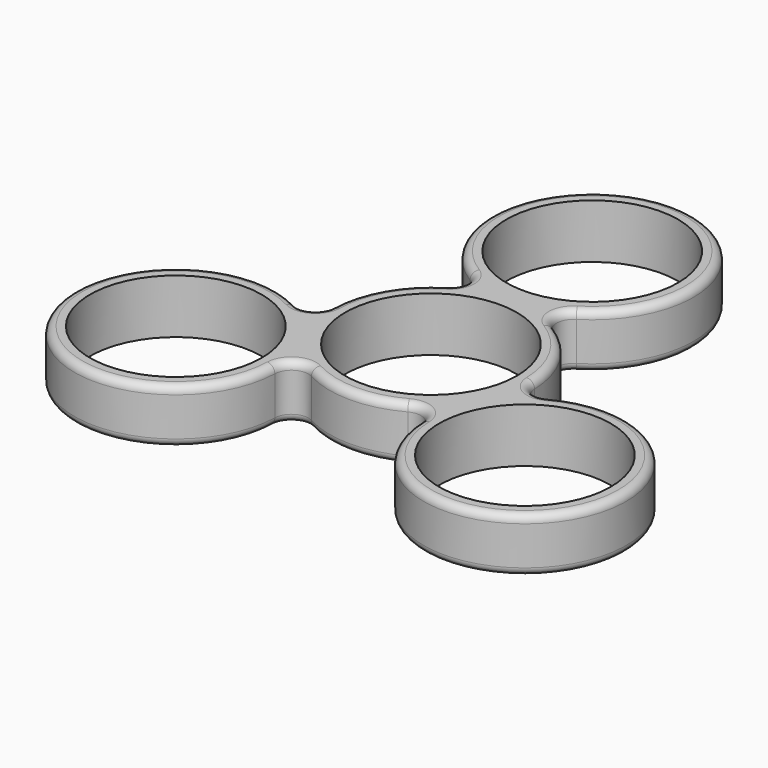
from build123d import *

# Parameters (mm, degrees)
F0_R     = 11.075
F1_DEPTH = 3.5
F2_R     = 1


# Not quite as in the source:
# - a feature names something its author has since deleted; it is built from what else it names


with BuildPart() as f1:
    # F0 (on Top) → F1 (new body, symmetric)
    with BuildSketch(Plane.XY):
        with BuildLine():
            ThreePointArc((6.8525738406, 11.1354324909), (0, 13.075), (-6.8525738406, 11.1354324909))
            ThreePointArc((-6.8525738406, 11.1354324909), (-11.3232821545, 6.5375), (-13.0698543395, 0.3667867818))
            ThreePointArc((-13.0698543395, 0.3667867818), (-11.3232821545, -6.5375), (-6.217280499, -11.5022192727))
            ThreePointArc((-6.217280499, -11.5022192727), (0, -13.075), (6.217280499, -11.5022192727))
            ThreePointArc((6.217280499, -11.5022192727), (8.3529990104, -11.5321813184), (9.4468061589, -13.3667867818))
            ThreePointArc((9.4468061589, -13.3667867818), (33.8399426529, -19.5375), (16.2993799994, -1.4977807273))
            ThreePointArc((16.2993799994, -1.4977807273), (14.163661488, -1.4678186816), (13.0698543395, 0.3667867818))
            ThreePointArc((13.0698543395, 0.3667867818), (11.3232821545, 6.5375), (6.8525738406, 11.1354324909))
        make_face()
        with Locations((22.5166604984, -13)):
            Circle(F0_R, mode=Mode.SUBTRACT)
        Circle(F0_R, mode=Mode.SUBTRACT)
        with BuildLine():
            ThreePointArc((-6.8525738406, 14.8645675091), (-5.8106624775, 13), (-6.8525738406, 11.1354324909))
            ThreePointArc((-6.8525738406, 11.1354324909), (0, 13.075), (6.8525738406, 11.1354324909))
            ThreePointArc((6.8525738406, 11.1354324909), (5.8106624775, 13), (6.8525738406, 14.8645675091))
            ThreePointArc((6.8525738406, 14.8645675091), (0, 39.075), (-6.8525738406, 14.8645675091))
        make_face()
        with Locations((0, 26)):
            Circle(F0_R, mode=Mode.SUBTRACT)
        with BuildLine():
            ThreePointArc((-6.217280499, -11.5022192727), (-11.3232821545, -6.5375), (-13.0698543395, 0.3667867818))
            ThreePointArc((-13.0698543395, 0.3667867818), (-14.163661488, -1.4678186816), (-16.2993799994, -1.4977807273))
            ThreePointArc((-16.2993799994, -1.4977807273), (-33.8399426529, -19.5375), (-9.4468061589, -13.3667867818))
            ThreePointArc((-9.4468061589, -13.3667867818), (-8.3529990104, -11.5321813184), (-6.217280499, -11.5022192727))
        make_face()
        with Locations((-22.5166604984, -13)):
            Circle(F0_R, mode=Mode.SUBTRACT)
    extrude(amount=F1_DEPTH, both=True)

    # F2
    f2_edges = [f1.edges().sort_by_distance(p)[0] for p in [
        (-14.163661, -1.467819, 3.5),
        (5.810662, 13, -3.5),
        (-5.810662, 13, 3.5),
        (-8.352999, -11.532181, 3.5),
        (5.810662, 13, 3.5),
        (-5.810662, 13, -3.5),
        (-14.163661, -1.467819, -3.5),
        (-8.352999, -11.532181, -3.5),
    ]]
    fillet(f2_edges, radius=F2_R)


solid = f1.part
